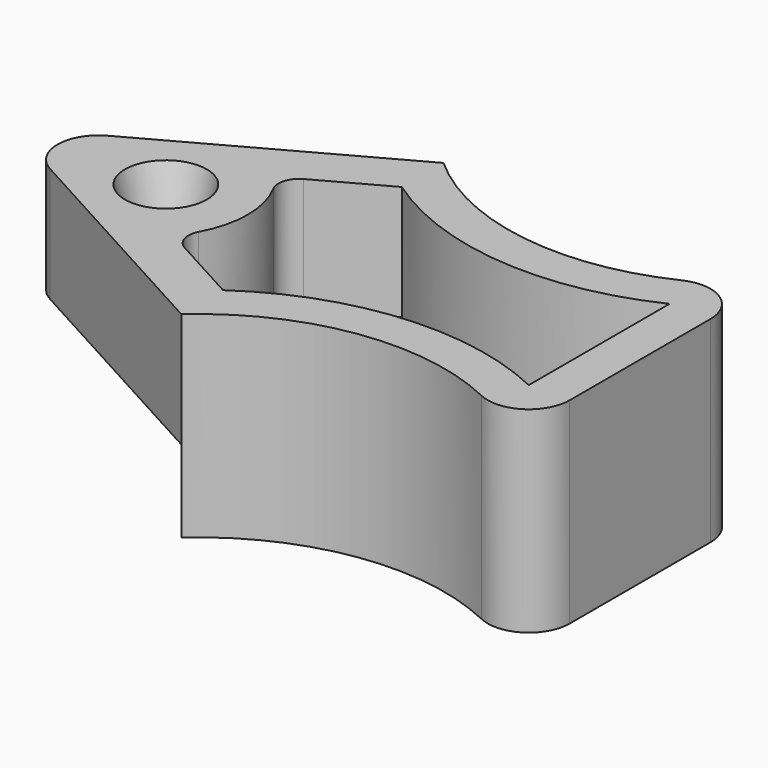
from build123d import *

# Parameters (mm, degrees)
F1_DEPTH = 15.24
F2_R     = 3.175
F5_DEPTH = 15.241
F6_W     = 38.1
F6_H     = 6.35
F7_DEPTH = 25.401


# Not quite as in the source:
# - an extrude whose draft closes it to a point is written as a loft to that point


with BuildPart() as f1:
    # F0 (on Top) → F1 (new body)
    with BuildSketch(Plane.XY):
        with BuildLine():
            ThreePointArc((-25.4, 25.4), (-53.7980633142, 12.7), (-25.4, 0))
            Line((-25.4, 0), (-34.5618496597, 0))
            Line((-34.5618496597, 0), (-34.5618496597, 25.4))
            Line((-34.5618496597, 25.4), (-25.4, 25.4))
        make_face()
        with BuildLine():
            Line((-34.5618496597, 0), (-25.4, 0))
            ThreePointArc((-25.4, 0), (-21.204965459, 5.7439235197), (-19.7203873372, 12.7))
            ThreePointArc((-19.7203873372, 12.7), (-21.204965459, 19.6560764803), (-25.4, 25.4))
            Line((-25.4, 25.4), (-34.5618496597, 25.4))
            Line((-34.5618496597, 25.4), (-34.5618496597, 0))
        make_face()
        with BuildLine():
            ThreePointArc((-19.7203873372, 12.7), (-21.204965459, 5.7439235197), (-25.4, 0))
            ThreePointArc((-25.4, 0), (-15.4225737421, 4.6554132358), (-4.5357142857, 3.0127938932))
            ThreePointArc((-4.5357142857, 3.0127938932), (-1.4778911139, 3.1980667262), (0, 5.8814314849))
            Line((0, 5.8814314849), (0, 19.5185685151))
            ThreePointArc((0, 19.5185685151), (-1.4778911139, 22.2019332738), (-4.5357142857, 22.3872061068))
            ThreePointArc((-4.5357142857, 22.3872061068), (-15.4225737421, 20.7445867642), (-25.4, 25.4))
            ThreePointArc((-25.4, 25.4), (-21.204965459, 19.6560764803), (-19.7203873372, 12.7))
        make_face()
    extrude(amount=F1_DEPTH)

    # F2 (on face) → F3 section 0
    with BuildSketch(Plane.XY.offset(15.24), mode=Mode.PRIVATE) as f3_s0:
        with Locations((-36.7592253257, 12.7)):
            Circle(F2_R)
    loft([f3_s0.sketch, Vertex(-36.7592253257, 12.7, 2.505770536)], ruled=True, mode=Mode.SUBTRACT)

    # F4 (on face) → F5 (cut, through all)
    with BuildSketch(Plane.XY.offset(15.24)):
        with BuildLine():
            ThreePointArc((-25.4, 4.0399547456), (-14.535188109, 7.9500701216), (-3.175, 5.8814314849))
            Line((-3.175, 5.8814314849), (-3.175, 19.5185685151))
            ThreePointArc((-3.175, 19.5185685151), (-14.535188109, 17.4499298784), (-25.4, 21.3600452544))
            Line((-25.4, 21.3600452544), (-30.6912422422, 18.4625566245))
            ThreePointArc((-30.6912422422, 18.4625566245), (-31.4514193427, 17.5192344091), (-31.3248088175, 16.3143710139))
            ThreePointArc((-31.3248088175, 16.3143710139), (-30.4092253257, 12.7), (-31.3248088175, 9.0856289861))
            ThreePointArc((-31.3248088175, 9.0856289861), (-31.4514193427, 7.8807655909), (-30.6912422422, 6.9374433755))
            Line((-30.6912422422, 6.9374433755), (-25.4, 4.0399547456))
        make_face()
        with BuildLine():
            ThreePointArc((-25.4, 25.4), (-53.7980633142, 12.7), (-25.4, 0))
            Line((-25.4, 0), (-43.5066161293, 9.9151979742))
            ThreePointArc((-43.5066161293, 9.9151979742), (-45.1566562358, 12.7), (-43.5066161293, 15.4848020258))
            Line((-43.5066161293, 15.4848020258), (-25.4, 25.4))
        make_face()
    extrude(amount=-F5_DEPTH, mode=Mode.SUBTRACT)

    # F6 (on Front) → F7 (cut, through all)
    with BuildSketch(Plane.XZ):
        with Locations((-44.45, 3.175)):
            Rectangle(F6_W, F6_H)
    extrude(amount=-F7_DEPTH, mode=Mode.SUBTRACT)


solid = f1.part
